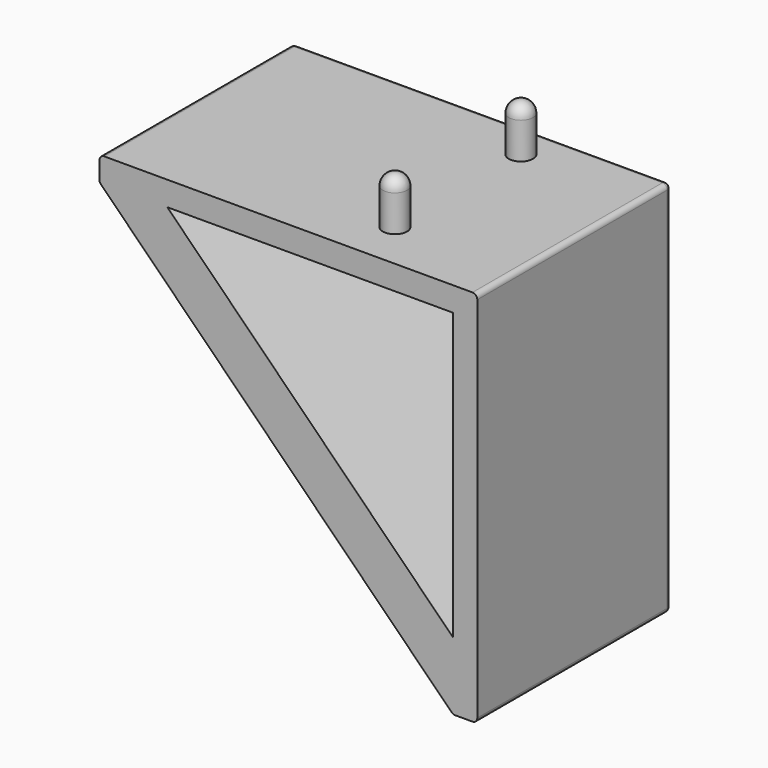
from build123d import *

# Parameters (mm, degrees)
F0_W           = 78
F0_H           = 50
F1_DEPTH       = 5
F2_R           = 2.5
F3_DEPTH       = 10
F4_R           = 2.5
F5_W           = 50
F5_H           = 78
F6_DEPTH       = 5
F8_DEPTH       = 50
F10_DEPTH      = 45
F11_T1_DEPTH   = 46.0355339059
F11_T3_DEPTH   = 92.6812408671
F11_T5_DEPTH   = 86.8528137424
F11_T7_DEPTH   = 76
F11_T9_DEPTH   = 76
F11_T11_DEPTH  = 3.5857864376
F11_T13_DEPTH  = 102.4091629285
F11_T15_DEPTH  = 3.5857864376
F11_T17_DEPTH  = 51.5
F11_T19_DEPTH  = 50.0355339059
F11_S23_W      = 1.02
F11_S23_H      = 1.02
F11_T24_DEPTH  = 1.02
F11_S29_W      = 1.02
F11_S29_H      = 1.02
F11_T30_DEPTH  = 1.02
F11_S35_W      = 1.02
F11_S35_H      = 1.02
F11_T36_DEPTH  = 1.02
F11_T42_DEPTH  = 1.02
F11_T48_DEPTH  = 1.02
F11_T54_DEPTH  = 61.5
F11_T59_DEPTH  = 61.5
F11_T64_DEPTH  = 88.43860018
F11_T70_DEPTH  = 103.9949493661
F11_T76_DEPTH  = 10.0857864376
F11_T81_DEPTH  = 10.0857864376
F11_T84_ANGLE  = 45
F11_T86_ANGLE  = 45
F11_T91_DEPTH  = 64
F11_T95_DEPTH  = 64
F11_T102_DEPTH = 61.5
F11_T106_DEPTH = 88.43860018
F11_T113_DEPTH = 61.5
F11_T117_DEPTH = 88.43860018
F11_T124_DEPTH = 10.0857864376
F11_T128_DEPTH = 103.9949493661
F11_T135_DEPTH = 103.9949493661
F11_T139_DEPTH = 10.0857864376


# Not quite as in the source:
# - a fillet or chamfer that OpenCascade refuses, or shapes differently, is made with other operations: its cross-section is extruded or revolved along the edge and cut away or added


with BuildPart() as f1:
    # F0 (on Top) → F1 (new body)
    with BuildSketch(Plane.XY):
        with Locations((12.5221835672, 0.070781447)):
            Rectangle(F0_W, F0_H)
    extrude(amount=F1_DEPTH)

    # F2 (on face) → F3 (join)
    with BuildSketch(Plane.XY.offset(5)):
        with Locations((26.5221835672, 17.570781447)):
            Circle(F2_R)
        with Locations((26.5221835672, -14.929218553)):
            Circle(F2_R)
    extrude(amount=F3_DEPTH)

    # F4
    f4_edges = [f1.edges().sort_by_distance(p)[0] for p in [
        (24.022184, 17.570781, 15),
        (24.022184, -14.929219, 15),
    ]]
    fillet(f4_edges, radius=F4_R)

    # F5 (on face) → F6 (join)
    with BuildSketch(Plane.YZ.offset(51.5221835672)):
        with Locations((0.070781447, -34)):
            Rectangle(F5_W, F5_H)
    extrude(amount=-F6_DEPTH)

    # F7 (on face) → F8 (join)
    with BuildSketch(Plane(origin=(0, 25.070781447, 0), x_dir=(-1, 0, 0), z_dir=(0, 1, 0))):
        Polygon((-46.5221835672, -73), (26.4778164328, 0), (12.4778164328, 0), (-46.5221835672, -59), align=None)
    extrude(amount=-F8_DEPTH)

    # F9 (on face) → F10 (cut)
    with BuildSketch(Plane(origin=(0, 25.070781447, 0), x_dir=(-1, 0, 0), z_dir=(0, 1, 0))):
        Polygon((15.4778164328, 0), (-46.5221835672, -62), (-46.5221835672, -70), (23.4778164328, 0), align=None)
    extrude(amount=-F10_DEPTH, mode=Mode.SUBTRACT)

    # F11: fillet of radius 1 on 20 edges, made by hand

    # F11_s2 → F11_t1 (join)
    with BuildSketch(Plane.XZ.offset(-25.070781447)):
        with BuildLine():
            ThreePointArc((-15.1849232139, -0.2928932188), (-15.5093465628, -0.0761204675), (-15.8920299951, 0))
            Line((-15.8920299951, 0), (-15.4778164328, 0))
            Line((-15.4778164328, 0), (-15.1849232139, -0.2928932188))
        make_face()
        with BuildLine():
            ThreePointArc((46.2292903484, -61.7071067812), (46.4460630998, -62.03153013), (46.5221835672, -62.4142135624))
            Line((46.5221835672, -62.4142135624), (46.5221835672, -62))
            Line((46.5221835672, -62), (46.2292903484, -61.7071067812))
        make_face()
    extrude(amount=F11_T1_DEPTH)

    # F11_s4 → F11_t3 (join)
    with BuildSketch(Plane(origin=(-9.5066751693, 0, 9.5066751693), x_dir=(0, 1, 0), z_dir=(0.7071067812, 0, -0.7071067812))):
        with BuildLine():
            ThreePointArc((-18.929218553, -10.9444689576), (-19.6363253342, -11.2373621764), (-19.929218553, -11.9444689576))
            Line((-19.929218553, -11.9444689576), (-19.929218553, -10.9444689576))
            Line((-19.929218553, -10.9444689576), (-18.929218553, -10.9444689576))
        make_face()
    extrude(amount=F11_T3_DEPTH)

    # F11_s6 → F11_t5 (cut)
    with BuildSketch(Plane(origin=(-7.4460149976, 0, 7.4460149976), x_dir=(0, 1, 0), z_dir=(0.7071067812, 0, -0.7071067812))):
        with BuildLine():
            ThreePointArc((25.070781447, -9.9444689576), (24.7778882282, -10.6515757388), (24.070781447, -10.9444689576))
            Line((24.070781447, -10.9444689576), (25.070781447, -10.9444689576))
            Line((25.070781447, -10.9444689576), (25.070781447, -9.9444689576))
        make_face()
    extrude(amount=F11_T5_DEPTH, mode=Mode.SUBTRACT)

    # F11_s8 → F11_t7 (cut)
    with BuildSketch(Plane.YZ.offset(-25.4778164328)):
        with BuildLine():
            ThreePointArc((24.070781447, 5), (24.7778882282, 4.7071067812), (25.070781447, 4))
            Line((25.070781447, 4), (25.070781447, 5))
            Line((25.070781447, 5), (24.070781447, 5))
        make_face()
    extrude(amount=F11_T7_DEPTH, mode=Mode.SUBTRACT)

    # F11_s10 → F11_t9 (cut)
    with BuildSketch(Plane.XY.offset(-72)):
        with BuildLine():
            ThreePointArc((51.5221835672, 24.070781447), (51.2292903484, 24.7778882282), (50.5221835672, 25.070781447))
            Line((50.5221835672, 25.070781447), (51.5221835672, 25.070781447))
            Line((51.5221835672, 25.070781447), (51.5221835672, 24.070781447))
        make_face()
    extrude(amount=F11_T9_DEPTH, mode=Mode.SUBTRACT)

    # F11_s12 → F11_t11 (cut)
    with BuildSketch(Plane.YZ.offset(46.9363971296)):
        with BuildLine():
            ThreePointArc((25.070781447, -72), (24.7778882282, -72.7071067812), (24.070781447, -73))
            Line((24.070781447, -73), (25.070781447, -73))
            Line((25.070781447, -73), (25.070781447, -72))
        make_face()
    extrude(amount=F11_T11_DEPTH, mode=Mode.SUBTRACT)

    # F11_s14 → F11_t13 (cut)
    with BuildSketch(Plane(origin=(59.4681985648, 0, -59.4681985648), x_dir=(0, 1, 0), z_dir=(-0.7071067812, 0, 0.7071067812))):
        with BuildLine():
            ThreePointArc((25.070781447, 17.7226435506), (24.7778882282, 18.4297503318), (24.070781447, 18.7226435506))
            Line((24.070781447, 18.7226435506), (25.070781447, 18.7226435506))
            Line((25.070781447, 18.7226435506), (25.070781447, 17.7226435506))
        make_face()
    extrude(amount=F11_T13_DEPTH, mode=Mode.SUBTRACT)

    # F11_s16 → F11_t15 (cut)
    with BuildSketch(Plane.XY.offset(0.4142135624)):
        with BuildLine():
            ThreePointArc((-25.4778164328, 25.070781447), (-26.1849232139, 24.7778882282), (-26.4778164328, 24.070781447))
            Line((-26.4778164328, 24.070781447), (-26.4778164328, 25.070781447))
            Line((-26.4778164328, 25.070781447), (-25.4778164328, 25.070781447))
        make_face()
    extrude(amount=F11_T15_DEPTH, mode=Mode.SUBTRACT)

    # F11_s18 → F11_t17 (cut)
    with BuildSketch(Plane.XZ.offset(-24.070781447)):
        with BuildLine():
            ThreePointArc((51.5221835672, -72), (51.2292903484, -72.7071067812), (50.5221835672, -73))
            Line((50.5221835672, -73), (51.5221835672, -73))
            Line((51.5221835672, -73), (51.5221835672, -72))
        make_face()
        with BuildLine():
            ThreePointArc((50.5221835672, 5), (51.2292903484, 4.7071067812), (51.5221835672, 4))
            Line((51.5221835672, 4), (51.5221835672, 5))
            Line((51.5221835672, 5), (50.5221835672, 5))
        make_face()
        with BuildLine():
            ThreePointArc((-25.4778164328, 5), (-26.1849232139, 4.7071067812), (-26.4778164328, 4))
            Line((-26.4778164328, 4), (-26.4778164328, 5))
            Line((-26.4778164328, 5), (-25.4778164328, 5))
        make_face()
    extrude(amount=F11_T17_DEPTH, mode=Mode.SUBTRACT)

    # F11_s20 → F11_t19 (cut)
    with BuildSketch(Plane.XZ.offset(-24.070781447)):
        with BuildLine():
            ThreePointArc((46.9363971296, -73), (46.5537136972, -72.9238795325), (46.2292903484, -72.7071067812))
            Line((46.2292903484, -72.7071067812), (46.5221835672, -73))
            Line((46.5221835672, -73), (46.9363971296, -73))
        make_face()
        with BuildLine():
            ThreePointArc((-26.4778164328, 0.4142135624), (-26.4016959653, 0.03153013), (-26.1849232139, -0.2928932188))
            Line((-26.1849232139, -0.2928932188), (-26.4778164328, 0))
            Line((-26.4778164328, 0), (-26.4778164328, 0.4142135624))
        make_face()
    extrude(amount=F11_T19_DEPTH, mode=Mode.SUBTRACT)


with BuildPart() as f11_tool22:
    # F11_s23 → F11_t24 (new body)
    with BuildSketch(Plane.XY.offset(4)):
        with Locations((51.0321835672, 24.580781447)):
            Rectangle(F11_S23_W, F11_S23_H)
    extrude(amount=F11_T24_DEPTH)

    # F11_s25 → F11_t26 (revolve, cut)
    with BuildSketch(Plane(origin=(50.5221835672, 24.070781447, 4), x_dir=(-0.7071067812, -0.7071067812, 0), z_dir=(-0.7071067812, 0.7071067812, 0))):
        with BuildLine():
            ThreePointArc((0, -1), (1, 0), (0, 1))
            Line((0, 1), (0, -1))
        make_face()
    revolve(axis=Axis((50.5221835672, 24.070781447, 4), (0, 0, 1)), mode=Mode.SUBTRACT)


with BuildPart() as f1_1:
    add(f1.part)

    # F11_t21: cut F11_tool22
    add(f11_tool22.part, mode=Mode.SUBTRACT)


with BuildPart() as f11_tool28:
    # F11_s29 → F11_t30 (new body)
    with BuildSketch(Plane.XY.offset(4)):
        with Locations((-25.9878164328, 24.580781447)):
            Rectangle(F11_S29_W, F11_S29_H)
    extrude(amount=F11_T30_DEPTH)

    # F11_s31 → F11_t32 (revolve, cut)
    with BuildSketch(Plane(origin=(-25.4778164328, 24.070781447, 4), x_dir=(0.7071067812, -0.7071067812, 0), z_dir=(-0.7071067812, -0.7071067812, 0))):
        with BuildLine():
            ThreePointArc((0, -1), (1, 0), (0, 1))
            Line((0, 1), (0, -1))
        make_face()
    revolve(axis=Axis((-25.4778164328, 24.070781447, 4), (0, 0, 1)), mode=Mode.SUBTRACT)


with BuildPart() as f1_2:
    add(f1_1.part)

    # F11_t27: cut F11_tool28
    add(f11_tool28.part, mode=Mode.SUBTRACT)


with BuildPart() as f11_tool34:
    # F11_s35 → F11_t36 (new body)
    with BuildSketch(Plane.XY.offset(-72)):
        with Locations((51.0321835672, 24.580781447)):
            Rectangle(F11_S35_W, F11_S35_H)
    extrude(amount=-F11_T36_DEPTH)

    # F11_s37 → F11_t38 (revolve, cut)
    with BuildSketch(Plane(origin=(50.5221835672, 24.070781447, -72), x_dir=(-0.7071067812, -0.7071067812, 0), z_dir=(0.7071067812, -0.7071067812, 0))):
        with BuildLine():
            ThreePointArc((0, -1), (1, 0), (0, 1))
            Line((0, 1), (0, -1))
        make_face()
    revolve(axis=Axis((50.5221835672, 24.070781447, -72), (0, 0, -1)), mode=Mode.SUBTRACT)


with BuildPart() as f1_3:
    add(f1_2.part)

    # F11_t33: cut F11_tool34
    add(f11_tool34.part, mode=Mode.SUBTRACT)


with BuildPart() as f11_tool40:
    # F11_s41 → F11_t42 (new body)
    with BuildSketch(Plane.XZ.offset(-24.070781447)):
        Polygon((46.9363971296, -72), (46.9363971296, -73.02), (46.513899296, -73.02), (46.2151482128, -72.7212489168), align=None)
    extrude(amount=-F11_T42_DEPTH)

    # F11_s43 → F11_t44 (revolve, cut)
    with BuildSketch(Plane(origin=(46.9363971296, 24.070781447, -72), x_dir=(0.3826834324, 0, 0.9238795325), z_dir=(-0.9238795325, 0, 0.3826834324))):
        with BuildLine():
            ThreePointArc((0, -1), (1, 0), (0, 1))
            Line((0, 1), (0, -1))
        make_face()
    revolve(axis=Axis((46.9363971296, 24.070781447, -72), (0, 1, 0)), mode=Mode.SUBTRACT)


with BuildPart() as f1_4:
    add(f1_3.part)

    # F11_t39: cut F11_tool40
    add(f11_tool40.part, mode=Mode.SUBTRACT)


with BuildPart() as f11_tool46:
    # F11_s47 → F11_t48 (new body)
    with BuildSketch(Plane.XZ.offset(-24.070781447)):
        Polygon((-25.4778164328, 0.4142135624), (-26.4978164328, 0.4142135624), (-26.4978164328, -0.0082842712), (-26.1990653496, -0.3070353544), align=None)
    extrude(amount=-F11_T48_DEPTH)

    # F11_s49 → F11_t50 (revolve, cut)
    with BuildSketch(Plane(origin=(-25.4778164328, 24.070781447, 0.4142135624), x_dir=(0.9238795325, 0, 0.3826834324), z_dir=(-0.3826834324, 0, 0.9238795325))):
        with BuildLine():
            ThreePointArc((0, -1), (1, 0), (0, 1))
            Line((0, 1), (0, -1))
        make_face()
    revolve(axis=Axis((-25.4778164328, 24.070781447, 0.4142135624), (0, 1, 0)), mode=Mode.SUBTRACT)


with BuildPart() as f1_5:
    add(f1_4.part)

    # F11_t45: cut F11_tool46
    add(f11_tool46.part, mode=Mode.SUBTRACT)


with BuildPart() as f11_tool52:
    # F11_s53 → F11_t54 (new body)
    with BuildSketch(Plane.YZ.offset(46.5221835672)):
        with BuildLine():
            ThreePointArc((25.070781447, 1), (24.7778882282, 0.2928932188), (24.070781447, 0))
            Line((24.070781447, 0), (25.070781447, 0))
            Line((25.070781447, 0), (25.070781447, 1))
        make_face()
    extrude(amount=-F11_T54_DEPTH)

    split(bisect_by=Plane(origin=(-6.2389082164, 0, -6.2389082164), x_dir=(0, 1, 0), z_dir=(0.7071067812, 0, 0.7071067812)), keep=Keep.TOP)


with BuildPart() as f1_6:
    add(f1_5.part)

    # F11_t51: cut F11_tool52
    add(f11_tool52.part, mode=Mode.SUBTRACT)


with BuildPart() as f11_tool57:
    # F11_s58 → F11_t59 (new body)
    with BuildSketch(Plane.XY.offset(-61.5)):
        with BuildLine():
            ThreePointArc((47.5221835672, 25.070781447), (46.8150767861, 24.7778882282), (46.5221835672, 24.070781447))
            Line((46.5221835672, 24.070781447), (46.5221835672, 25.070781447))
            Line((46.5221835672, 25.070781447), (47.5221835672, 25.070781447))
        make_face()
    extrude(amount=F11_T59_DEPTH)

    split(bisect_by=Plane(origin=(-6.2389082164, 0, -6.2389082164), x_dir=(0, 1, 0), z_dir=(0.7071067812, 0, 0.7071067812)), keep=Keep.TOP)


with BuildPart() as f1_7:
    add(f1_6.part)

    # F11_t56: cut F11_tool57
    add(f11_tool57.part, mode=Mode.SUBTRACT)


with BuildPart() as f11_tool62:
    # F11_s63 → F11_t64 (new body)
    with BuildSketch(Plane(origin=(-8.0066751693, 0, 8.0066751693), x_dir=(0, 1, 0), z_dir=(0.7071067812, 0, -0.7071067812))):
        with BuildLine():
            ThreePointArc((25.070781447, -9.823148614), (24.7778882282, -9.1160418328), (24.070781447, -8.823148614))
            Line((24.070781447, -8.823148614), (25.070781447, -8.823148614))
            Line((25.070781447, -8.823148614), (25.070781447, -9.823148614))
        make_face()
    extrude(amount=F11_T64_DEPTH)

    split(bisect_by=Plane.XY, keep=Keep.BOTTOM)

    split(bisect_by=Plane.YZ.offset(46.5221835672), keep=Keep.BOTTOM)


with BuildPart() as f1_8:
    add(f1_7.part)

    # F11_t61: cut F11_tool62
    add(f11_tool62.part, mode=Mode.SUBTRACT)


with BuildPart() as f11_tool68:
    # F11_s69 → F11_t70 (new body)
    with BuildSketch(Plane(origin=(60.0288587366, 0, -60.0288587366), x_dir=(0, 1, 0), z_dir=(-0.7071067812, 0, 0.7071067812))):
        with BuildLine():
            ThreePointArc((25.070781447, 17.6013232071), (24.7778882282, 16.8942164259), (24.070781447, 16.6013232071))
            Line((24.070781447, 16.6013232071), (25.070781447, 16.6013232071))
            Line((25.070781447, 16.6013232071), (25.070781447, 17.6013232071))
        make_face()
    extrude(amount=F11_T70_DEPTH)

    split(bisect_by=Plane.XY, keep=Keep.BOTTOM)

    split(bisect_by=Plane.YZ.offset(46.5221835672), keep=Keep.BOTTOM)


with BuildPart() as f1_9:
    add(f1_8.part)

    # F11_t67: cut F11_tool68
    add(f11_tool68.part, mode=Mode.SUBTRACT)


with BuildPart() as f11_tool74:
    # F11_s75 → F11_t76 (new body)
    with BuildSketch(Plane.YZ.offset(-25.9778164328)):
        with BuildLine():
            ThreePointArc((25.070781447, 1), (24.7778882282, 0.2928932188), (24.070781447, 0))
            Line((24.070781447, 0), (25.070781447, 0))
            Line((25.070781447, 0), (25.070781447, 1))
        make_face()
    extrude(amount=F11_T76_DEPTH)

    split(bisect_by=Plane(origin=(-11.7389082164, 0, -11.7389082164), x_dir=(0, 1, 0), z_dir=(0.7071067812, 0, 0.7071067812)), keep=Keep.TOP)


with BuildPart() as f1_10:
    add(f1_9.part)

    # F11_t73: cut F11_tool74
    add(f11_tool74.part, mode=Mode.SUBTRACT)


with BuildPart() as f11_tool79:
    # F11_s80 → F11_t81 (new body)
    with BuildSketch(Plane.XY.offset(-62.4142135624)):
        with BuildLine():
            ThreePointArc((47.5221835672, 25.070781447), (46.8150767861, 24.7778882282), (46.5221835672, 24.070781447))
            Line((46.5221835672, 24.070781447), (46.5221835672, 25.070781447))
            Line((46.5221835672, 25.070781447), (47.5221835672, 25.070781447))
        make_face()
    extrude(amount=-F11_T81_DEPTH)

    split(bisect_by=Plane(origin=(-11.7389082164, 0, -11.7389082164), x_dir=(0, 1, 0), z_dir=(0.7071067812, 0, 0.7071067812)), keep=Keep.TOP)


with BuildPart() as f1_11:
    add(f1_10.part)

    # F11_t78: cut F11_tool79
    add(f11_tool79.part, mode=Mode.SUBTRACT)

    # F11_s83 → F11_t84 (revolve, cut)
    with BuildSketch(Plane(origin=(53.9681985648, 0, -53.9681985648), x_dir=(0, 1, 0), z_dir=(-0.7071067812, 0, 0.7071067812))):
        with BuildLine():
            ThreePointArc((25.070781447, 9.9444689576), (24.7778882282, 10.6515757388), (24.070781447, 10.9444689576))
            Line((24.070781447, 10.9444689576), (25.070781447, 10.9444689576))
            Line((25.070781447, 10.9444689576), (25.070781447, 9.9444689576))
        make_face()
    revolve(axis=Axis((45.5221835672, 25.070781447, -62.4142135624), (0, 1, 0)), revolution_arc=F11_T84_ANGLE, mode=Mode.SUBTRACT)

    # F11_s85 → F11_t86 (revolve, cut)
    with BuildSketch(Plane(origin=(-7.4460149976, 0, 7.4460149976), x_dir=(0, 1, 0), z_dir=(0.7071067812, 0, -0.7071067812))):
        with BuildLine():
            ThreePointArc((25.070781447, -9.9444689576), (24.7778882282, -10.6515757388), (24.070781447, -10.9444689576))
            Line((24.070781447, -10.9444689576), (25.070781447, -10.9444689576))
            Line((25.070781447, -10.9444689576), (25.070781447, -9.9444689576))
        make_face()
    revolve(axis=Axis((-15.8920299951, 25.070781447, -1), (0, -1, 0)), revolution_arc=F11_T86_ANGLE, mode=Mode.SUBTRACT)


with BuildPart() as f11_tool89:
    # F11_s90 → F11_t91 (new body)
    with BuildSketch(Plane.YZ.offset(49.0221835672)):
        with BuildLine():
            ThreePointArc((25.070781447, 1), (24.7778882282, 0.2928932188), (24.070781447, 0))
            Line((24.070781447, 0), (25.070781447, 0))
            Line((25.070781447, 0), (25.070781447, 1))
        make_face()
    extrude(amount=-F11_T91_DEPTH)

    split(bisect_by=Plane.YZ.offset(46.5221835672), keep=Keep.TOP)


with BuildPart() as f11_tool93:
    # F11_s94 → F11_t95 (new body)
    with BuildSketch(Plane.XY.offset(-61.5)):
        with BuildLine():
            ThreePointArc((47.5221835672, 25.070781447), (46.8150767861, 24.7778882282), (46.5221835672, 24.070781447))
            Line((46.5221835672, 24.070781447), (46.5221835672, 25.070781447))
            Line((46.5221835672, 25.070781447), (47.5221835672, 25.070781447))
        make_face()
    extrude(amount=F11_T95_DEPTH)

    split(bisect_by=Plane.XY, keep=Keep.TOP)


with BuildPart() as f11_tool89_1:
    add(f11_tool89.part)

    # F11_t97: intersect F11_tool93
    add(f11_tool93.part, mode=Mode.INTERSECT)


with BuildPart() as f1_12:
    add(f1_11.part)

    # F11_t87: cut F11_tool89
    add(f11_tool89_1.part, mode=Mode.SUBTRACT)


with BuildPart() as f11_tool100:
    # F11_s101 → F11_t102 (new body)
    with BuildSketch(Plane.YZ.offset(46.5221835672)):
        with BuildLine():
            ThreePointArc((25.070781447, 1), (24.7778882282, 0.2928932188), (24.070781447, 0))
            Line((24.070781447, 0), (25.070781447, 0))
            Line((25.070781447, 0), (25.070781447, 1))
        make_face()
    extrude(amount=-F11_T102_DEPTH)

    split(bisect_by=Plane(origin=(-6.2389082164, 0, -6.2389082164), x_dir=(0, 1, 0), z_dir=(-0.7071067812, 0, -0.7071067812)), keep=Keep.TOP)


with BuildPart() as f11_tool104:
    # F11_s105 → F11_t106 (new body)
    with BuildSketch(Plane(origin=(-8.0066751693, 0, 8.0066751693), x_dir=(0, 1, 0), z_dir=(0.7071067812, 0, -0.7071067812))):
        with BuildLine():
            ThreePointArc((25.070781447, -9.823148614), (24.7778882282, -9.1160418328), (24.070781447, -8.823148614))
            Line((24.070781447, -8.823148614), (25.070781447, -8.823148614))
            Line((25.070781447, -8.823148614), (25.070781447, -9.823148614))
        make_face()
    extrude(amount=F11_T106_DEPTH)

    split(bisect_by=Plane.XY, keep=Keep.TOP)


with BuildPart() as f11_tool100_1:
    add(f11_tool100.part)

    # F11_t108: intersect F11_tool104
    add(f11_tool104.part, mode=Mode.INTERSECT)


with BuildPart() as f1_13:
    add(f1_12.part)

    # F11_t98: cut F11_tool100
    add(f11_tool100_1.part, mode=Mode.SUBTRACT)


with BuildPart() as f11_tool111:
    # F11_s112 → F11_t113 (new body)
    with BuildSketch(Plane.XY.offset(-61.5)):
        with BuildLine():
            ThreePointArc((47.5221835672, 25.070781447), (46.8150767861, 24.7778882282), (46.5221835672, 24.070781447))
            Line((46.5221835672, 24.070781447), (46.5221835672, 25.070781447))
            Line((46.5221835672, 25.070781447), (47.5221835672, 25.070781447))
        make_face()
    extrude(amount=F11_T113_DEPTH)

    split(bisect_by=Plane(origin=(-6.2389082164, 0, -6.2389082164), x_dir=(0, 1, 0), z_dir=(-0.7071067812, 0, -0.7071067812)), keep=Keep.TOP)


with BuildPart() as f11_tool115:
    # F11_s116 → F11_t117 (new body)
    with BuildSketch(Plane(origin=(-8.0066751693, 0, 8.0066751693), x_dir=(0, 1, 0), z_dir=(0.7071067812, 0, -0.7071067812))):
        with BuildLine():
            ThreePointArc((25.070781447, -9.823148614), (24.7778882282, -9.1160418328), (24.070781447, -8.823148614))
            Line((24.070781447, -8.823148614), (25.070781447, -8.823148614))
            Line((25.070781447, -8.823148614), (25.070781447, -9.823148614))
        make_face()
    extrude(amount=F11_T117_DEPTH)

    split(bisect_by=Plane.YZ.offset(46.5221835672), keep=Keep.TOP)


with BuildPart() as f11_tool111_1:
    add(f11_tool111.part)

    # F11_t119: intersect F11_tool115
    add(f11_tool115.part, mode=Mode.INTERSECT)


with BuildPart() as f1_14:
    add(f1_13.part)

    # F11_t109: cut F11_tool111
    add(f11_tool111_1.part, mode=Mode.SUBTRACT)


with BuildPart() as f11_tool122:
    # F11_s123 → F11_t124 (new body)
    with BuildSketch(Plane.XY.offset(-62.4142135624)):
        with BuildLine():
            ThreePointArc((47.5221835672, 25.070781447), (46.8150767861, 24.7778882282), (46.5221835672, 24.070781447))
            Line((46.5221835672, 24.070781447), (46.5221835672, 25.070781447))
            Line((46.5221835672, 25.070781447), (47.5221835672, 25.070781447))
        make_face()
    extrude(amount=-F11_T124_DEPTH)

    split(bisect_by=Plane(origin=(-11.7389082164, 0, -11.7389082164), x_dir=(0, 1, 0), z_dir=(-0.7071067812, 0, -0.7071067812)), keep=Keep.TOP)


with BuildPart() as f11_tool126:
    # F11_s127 → F11_t128 (new body)
    with BuildSketch(Plane(origin=(60.0288587366, 0, -60.0288587366), x_dir=(0, 1, 0), z_dir=(-0.7071067812, 0, 0.7071067812))):
        with BuildLine():
            ThreePointArc((25.070781447, 17.6013232071), (24.7778882282, 16.8942164259), (24.070781447, 16.6013232071))
            Line((24.070781447, 16.6013232071), (25.070781447, 16.6013232071))
            Line((25.070781447, 16.6013232071), (25.070781447, 17.6013232071))
        make_face()
    extrude(amount=F11_T128_DEPTH)

    split(bisect_by=Plane.YZ.offset(46.5221835672), keep=Keep.TOP)


with BuildPart() as f11_tool122_1:
    add(f11_tool122.part)

    # F11_t130: intersect F11_tool126
    add(f11_tool126.part, mode=Mode.INTERSECT)


with BuildPart() as f1_15:
    add(f1_14.part)

    # F11_t120: cut F11_tool122
    add(f11_tool122_1.part, mode=Mode.SUBTRACT)


with BuildPart() as f11_tool133:
    # F11_s134 → F11_t135 (new body)
    with BuildSketch(Plane(origin=(60.0288587366, 0, -60.0288587366), x_dir=(0, 1, 0), z_dir=(-0.7071067812, 0, 0.7071067812))):
        with BuildLine():
            ThreePointArc((25.070781447, 17.6013232071), (24.7778882282, 16.8942164259), (24.070781447, 16.6013232071))
            Line((24.070781447, 16.6013232071), (25.070781447, 16.6013232071))
            Line((25.070781447, 16.6013232071), (25.070781447, 17.6013232071))
        make_face()
    extrude(amount=F11_T135_DEPTH)

    split(bisect_by=Plane.XY, keep=Keep.TOP)


with BuildPart() as f11_tool137:
    # F11_s138 → F11_t139 (new body)
    with BuildSketch(Plane.YZ.offset(-25.9778164328)):
        with BuildLine():
            ThreePointArc((25.070781447, 1), (24.7778882282, 0.2928932188), (24.070781447, 0))
            Line((24.070781447, 0), (25.070781447, 0))
            Line((25.070781447, 0), (25.070781447, 1))
        make_face()
    extrude(amount=F11_T139_DEPTH)

    split(bisect_by=Plane(origin=(-11.7389082164, 0, -11.7389082164), x_dir=(0, 1, 0), z_dir=(-0.7071067812, 0, -0.7071067812)), keep=Keep.TOP)


with BuildPart() as f11_tool133_1:
    add(f11_tool133.part)

    # F11_t141: intersect F11_tool137
    add(f11_tool137.part, mode=Mode.INTERSECT)


with BuildPart() as f1_16:
    add(f1_15.part)

    # F11_t131: cut F11_tool133
    add(f11_tool133_1.part, mode=Mode.SUBTRACT)


solid = f1_16.part
